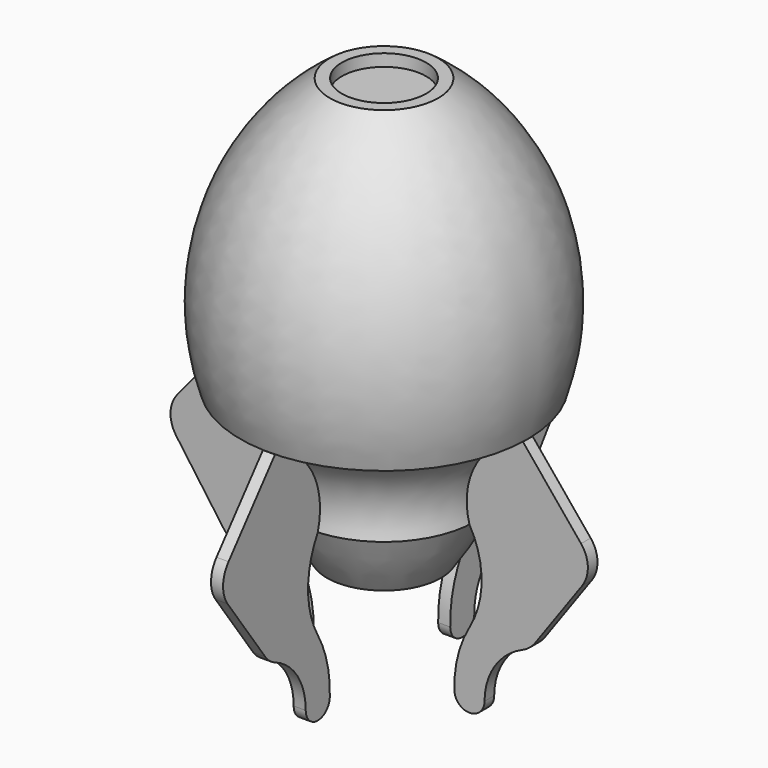
from build123d import *

# Parameters (mm, degrees)
F3_DEPTH        = 1
F3_COPIES_COUNT = 4
F4_R            = 10
F5_DEPTH        = 10


# Not quite as in the source:
# - a pattern or mirror of a feature is missing from the dataset's text; its kind, count and spacing are read off the source's solid


with BuildPart() as f1:
    # F0 (on Front) → F1 (revolve)
    with BuildSketch(Plane.XZ):
        with BuildLine():
            Line((0, 20), (0, 0))
            ThreePointArc((0, 0), (8.7701665379, 9.0473750966), (15, 20))
            Line((15, 20), (0, 20))
        make_face()
        with BuildLine():
            Line((0, 35), (0, 20))
            Line((0, 20), (15, 20))
            ThreePointArc((15, 20), (16.2110312428, 29.4105971201), (23.8781369728, 35))
            Line((23.8781369728, 35), (0, 35))
        make_face()
        with BuildLine():
            Line((0, 78), (0, 35))
            Line((0, 35), (23.8781369728, 35))
            ThreePointArc((23.8781369728, 35), (23.8216511077, 59.9408683434), (9, 80))
            Line((9, 80), (7, 80))
            Line((7, 80), (7, 78))
            Line((7, 78), (0, 78))
        make_face()
    revolve(axis=Axis((0, 0, 40), (0, 0, 1)))

    # F4 (on Top) → F5 (cut)
    with BuildSketch(Plane.XY):
        Circle(F4_R)
    extrude(amount=F5_DEPTH, mode=Mode.SUBTRACT)


with BuildPart() as f3:
    # F2 (on Front) → F3 (new body, symmetric)
    with BuildSketch(Plane.XZ):
        with BuildLine():
            Line((-23.8781369728, 35), (-15, 20))
            ThreePointArc((-15, 20), (-16.2110312428, 29.4105971201), (-23.8781369728, 35))
        make_face()
        with BuildLine():
            ThreePointArc((-15, 5), (-17.0096189432, 12.5), (-15, 20))
            Line((-15, 20), (-23.8781369728, 35))
            Line((-23.8781369728, 35), (-33.5194520938, 23.2540039676))
            ThreePointArc((-33.5194520938, 23.2540039676), (-34.6519714837, 20.2457265839), (-33.7191362857, 17.1696655509))
            Line((-33.7191362857, 17.1696655509), (-25.8983518836, 6.2538675406))
            ThreePointArc((-25.8983518836, 6.2538675406), (-25.3056790569, 5.5677822491), (-24.598856997, 5))
            Line((-24.598856997, 5), (-15, 5))
        make_face()
        with BuildLine():
            ThreePointArc((-12.5, -5), (-13.0489084102, 0.1752728974), (-15, 5))
            Line((-15, 5), (-15, -5))
            Line((-15, -5), (-12.5, -5))
        make_face()
        with BuildLine():
            Line((-15, -5), (-15, 5))
            Line((-15, 5), (-24.598856997, 5))
            ThreePointArc((-24.598856997, 5), (-24.2124315162, 4.7679111648), (-23.8066741128, 4.571567565))
            ThreePointArc((-23.8066741128, 4.571567565), (-19.2184091722, 0.7312530047), (-17.5, -5))
            Line((-17.5, -5), (-15, -5))
        make_face()
        with BuildLine():
            Line((-12.5, -5), (-15, -5))
            Line((-15, -5), (-17.5, -5))
            ThreePointArc((-17.5, -5), (-15, -7.5), (-12.5, -5))
        make_face()
    extrude(amount=F3_DEPTH, both=True)


with BuildPart() as f3_copies_1:
    # F3_copies: instance of F3
    add(f3.part.rotate(Axis((0, 0, 0), (0, 0, 1)), 1 * 360 / F3_COPIES_COUNT))


with BuildPart() as f3_copies_2:
    # F3_copies: instance of F3
    add(f3.part.rotate(Axis((0, 0, 0), (0, 0, 1)), 2 * 360 / F3_COPIES_COUNT))


with BuildPart() as f3_copies_3:
    # F3_copies: instance of F3
    add(f3.part.rotate(Axis((0, 0, 0), (0, 0, 1)), 3 * 360 / F3_COPIES_COUNT))


solid = Compound([f1.part, f3.part, f3_copies_1.part, f3_copies_2.part, f3_copies_3.part])
